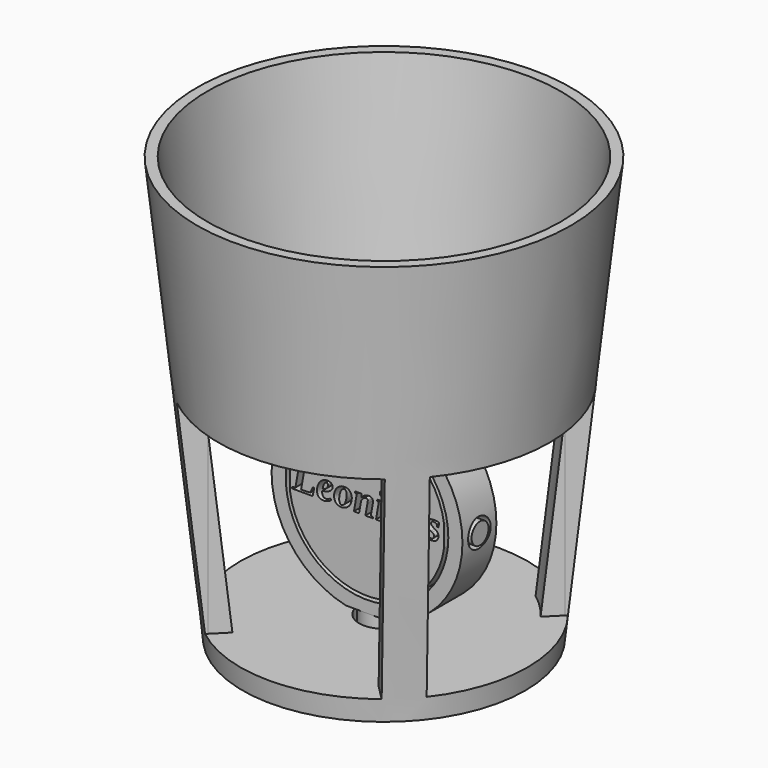
from build123d import *

# Parameters (mm, degrees)
F3_DEPTH      = 29
F4_R          = 3.5
F5_DEPTH      = 2
F5_DEPTH_BACK = 31
F6_R          = 11.5
F7_DEPTH      = 3
F8_R          = 2
F9_DEPTH      = 15
F11_DEPTH     = 3
F16_TEXT_SIZE = 5.5555555556
F17_DEPTH     = 2
F18_TEXT_SIZE = 7.6388888889
F19_DEPTH     = 2


# Not quite as in the source:
# - Text() gives the source's letters only with a copy of the font that has no kerning and outlines rounded to 1/6400 em; it was checked with that copy


with BuildPart() as f1:
    # F0 (on Front) → F1 (revolve)
    with BuildSketch(Plane.XZ):
        Polygon((0, 3), (0, 0), (20, 0), (26.4482922192, 60), (25, 60), (22.3132115753, 35), (0, 35), (0, 32), (20.4218137269, 32), (17.3051391543, 3), align=None)
    revolve(axis=Axis((0, 0, 33.5), (0, 0, 1)))

    # F2 (on face) → F3 (cut)
    with BuildSketch(Plane.XY.offset(3)):
        with BuildLine():
            Line((12.2634482474, 15.7989821534), (15.6845353346, 19.2200692405))
            ThreePointArc((15.6845353346, 19.2200692405), (0, 24.8075736474), (-15.6845353346, 19.2200692405))
            Line((-15.6845353346, 19.2200692405), (-12.2634482474, 15.7989821534))
            Line((-12.2634482474, 15.7989821534), (-8.6904833787, 12.2260172846))
            ThreePointArc((-8.6904833787, 12.2260172846), (0, 15), (8.6904833787, 12.2260172846))
            Line((8.6904833787, 12.2260172846), (12.2634482474, 15.7989821534))
        make_face()
        with BuildLine():
            Line((19.2200692405, 15.6845353346), (15.7989821534, 12.2634482474))
            Line((15.7989821534, 12.2634482474), (12.2260172846, 8.6904833787))
            ThreePointArc((12.2260172846, 8.6904833787), (15, 0), (12.2260172846, -8.6904833787))
            Line((12.2260172846, -8.6904833787), (15.7989821534, -12.2634482474))
            Line((15.7989821534, -12.2634482474), (19.2200692405, -15.6845353346))
            ThreePointArc((19.2200692405, -15.6845353346), (24.8075736474, 0), (19.2200692405, 15.6845353346))
        make_face()
        with BuildLine():
            Line((-12.2260172846, 8.6904833787), (-15.7989821534, 12.2634482474))
            Line((-15.7989821534, 12.2634482474), (-19.2200692405, 15.6845353346))
            ThreePointArc((-19.2200692405, 15.6845353346), (-24.8075736474, 0), (-19.2200692405, -15.6845353346))
            Line((-19.2200692405, -15.6845353346), (-15.7989821534, -12.2634482474))
            Line((-15.7989821534, -12.2634482474), (-12.2260172846, -8.6904833787))
            ThreePointArc((-12.2260172846, -8.6904833787), (-15, 0), (-12.2260172846, 8.6904833787))
        make_face()
        with BuildLine():
            Line((15.6845353346, -19.2200692405), (12.2634482474, -15.7989821534))
            Line((12.2634482474, -15.7989821534), (8.6904833787, -12.2260172846))
            ThreePointArc((8.6904833787, -12.2260172846), (0, -15), (-8.6904833787, -12.2260172846))
            Line((-8.6904833787, -12.2260172846), (-12.2634482474, -15.7989821534))
            Line((-12.2634482474, -15.7989821534), (-15.6845353346, -19.2200692405))
            ThreePointArc((-15.6845353346, -19.2200692405), (0, -24.8075736474), (15.6845353346, -19.2200692405))
        make_face()
    extrude(amount=F3_DEPTH, mode=Mode.SUBTRACT)

    # F4 (on face) → F5 (cut, two sides)
    with BuildSketch(Plane.XY.offset(3)) as f5_sk:
        Circle(F4_R)
    extrude(amount=-F5_DEPTH, mode=Mode.SUBTRACT)
    extrude(f5_sk.sketch, amount=F5_DEPTH_BACK, mode=Mode.SUBTRACT)


with BuildPart() as f7:
    # F6 (on Front) → F7 (new body, symmetric)
    with BuildSketch(Plane.XZ):
        with BuildLine():
            Line((3, 33.25), (0, 33.25))
            Line((0, 33.25), (-3, 33.25))
            Line((-3, 33.25), (-3, 30.6624465811))
            ThreePointArc((-3, 30.6624465811), (-13.5, 17.5), (-3, 4.3375534189))
            Line((-3, 4.3375534189), (-3, 1.75))
            Line((-3, 1.75), (0, 1.75))
            Line((0, 1.75), (3, 1.75))
            Line((3, 1.75), (3, 4.3375534189))
            ThreePointArc((3, 4.3375534189), (13.5, 17.5), (3, 30.6624465811))
            Line((3, 30.6624465811), (3, 33.25))
        make_face()
        with Locations((0, 17.5)):
            Circle(F6_R, mode=Mode.SUBTRACT)
    extrude(amount=F7_DEPTH, both=True)

    # F8 (on Right) → F9 (cut, symmetric)
    with BuildSketch(Plane.YZ):
        with Locations((0, 17.5)):
            Circle(F8_R)
    extrude(amount=F9_DEPTH, both=True, mode=Mode.SUBTRACT)

    # F12 (on Front) → F13 (revolve, cut)
    with BuildSketch(Plane.XZ):
        Polygon((0, 33.25), (3, 33.25), (3, 30.6624465811), (5, 30.6624465811), (5, 34.3002825975), (0, 34.3002825975), align=None)
        Polygon((5, 0.6997174025), (5, 4.3375534189), (3, 4.3375534189), (3, 1.75), (0, 1.75), (0, 0.6997174025), align=None)
    revolve(axis=Axis((0, 0, 33.7751412988), (0, 0, 1)), mode=Mode.SUBTRACT)


with BuildPart() as f11:
    # F10 (on Front) → F11 (new body, symmetric)
    with BuildSketch(Plane.XZ):
        with BuildLine():
            Line((13.5883981235, 19), (10.8972473589, 19))
            ThreePointArc((10.8972473589, 19), (0, 28.5), (-10.8972473589, 19))
            Line((-10.8972473589, 19), (-13.5883981235, 19))
            Line((-13.5883981235, 19), (-13.5883981235, 17.5))
            Line((-13.5883981235, 17.5), (-13.5883981235, 16))
            Line((-13.5883981235, 16), (-10.8972473589, 16))
            ThreePointArc((-10.8972473589, 16), (0, 6.5), (10.8972473589, 16))
            Line((10.8972473589, 16), (13.5883981235, 16))
            Line((13.5883981235, 16), (13.5883981235, 17.5))
            Line((13.5883981235, 17.5), (13.5883981235, 19))
        make_face()
    extrude(amount=F11_DEPTH, both=True)

    # F14 (on Front) → F15 (revolve, cut)
    with BuildSketch(Plane.XZ):
        Polygon((10.8972473589, 22.3522800952), (10.8972473589, 19), (13.5883981235, 19), (13.5883981235, 17.5), (14.9963386357, 17.5), (14.9963386357, 22.3522800952), align=None)
        Polygon((-14.9963386357, 17.5), (-13.5883981235, 17.5), (-13.5883981235, 19), (-10.8972473589, 19), (-10.8972473589, 22.3522800952), (-14.9963386357, 22.3522800952), align=None)
    revolve(axis=Axis((-14.2923683796, 0, 17.5), (1, 0, 0)), mode=Mode.SUBTRACT)

    # F16 (on face) → F17 (cut)
    with BuildSketch(Plane.XZ.offset(3)):
        with Locations((-10.6024305556, 16.4306085229)):
            Text('Leonidas', F16_TEXT_SIZE, font='Tinos', font_style=FontStyle.BOLDITALIC, text_align=(TextAlign.LEFT, TextAlign.BOTTOM))
    extrude(amount=-F17_DEPTH, mode=Mode.SUBTRACT)

    # F18 (on face) → F19 (cut)
    with BuildSketch(Plane(origin=(0, 3, 0), x_dir=(-1, 0, 0), z_dir=(0, 1, 0))):
        with Locations((-4.2318250868, 20.9452674775)):
            Text('21', F18_TEXT_SIZE, font='Tinos', font_style=FontStyle.BOLDITALIC, text_align=(TextAlign.LEFT, TextAlign.BOTTOM))
        with Locations((-8.0512695313, 12.1605452552)):
            Text('2017', F18_TEXT_SIZE, font='Tinos', font_style=FontStyle.BOLDITALIC, text_align=(TextAlign.LEFT, TextAlign.BOTTOM))
    extrude(amount=-F19_DEPTH, mode=Mode.SUBTRACT)


solid = Compound([f1.part, f7.part, f11.part])
